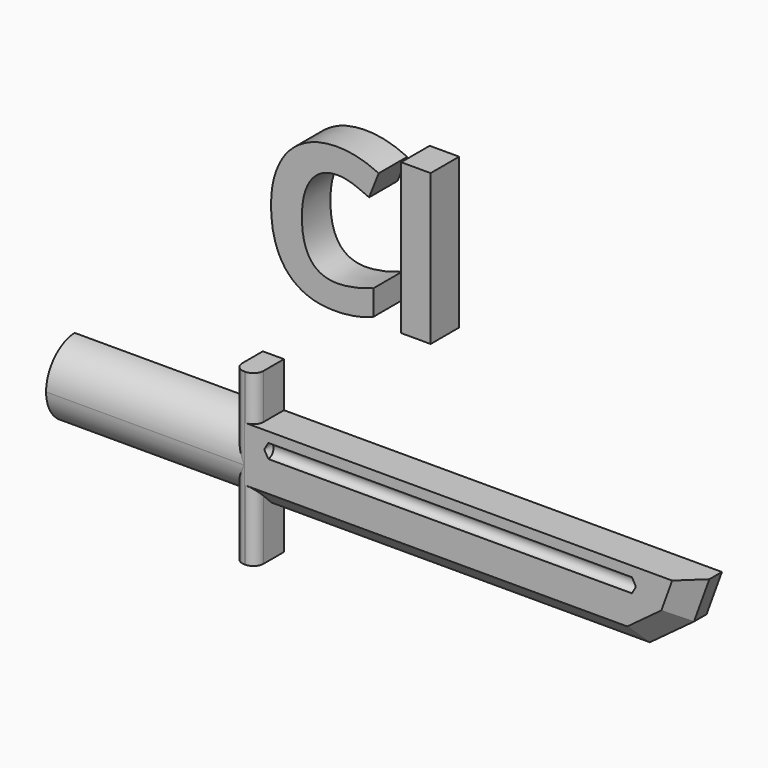
from build123d import *

# Parameters (mm, degrees)
F0_W         = 33.5415452719
F0_H         = 13.3481640369
F0_TEXT_SIZE = 35.2777777778
F1_DEPTH     = 6.35
F2_T1_DEPTH  = 50.2216307033
F3_SIZE      = 3.556
F5_D         = 2.54
F5_DEPTH     = 50.8
F5_TIP       = 0.7630929862
F6_D         = 2.54
F6_DEPTH     = 13.97
F6_TIP       = 0.7630929862
F7_R         = 1.778


# Not quite as in the source:
# - a fillet or chamfer that OpenCascade refuses, or shapes differently, is made with other operations: its cross-section is extruded or revolved along the edge and cut away or added
# - Text() gives the source's letters only with a copy of the font that has no kerning and outlines rounded to 1/6400 em; it was checked with that copy


with BuildPart() as f1:
    # F0 (on Front) → F1 (new body)
    with BuildSketch(Plane.XZ):
        with Locations((-36.8084944785, -14.685629867)):
            Rectangle(F0_W, F0_H)
        Polygon((-20.0377218425, 0), (-20.0377218425, -8.0115478486), (-20.0377218425, -21.3597118855), (-20.0377218425, -30.2584897727), (-16.2728521973, -30.2584897727), (-16.2728521973, -21.3597118855), (-16.2728521973, -11.7764146999), (-16.2728521973, -8.0115478486), (-16.2728521973, 0), align=None)
        Polygon((61.7625713348, -8.0115478486), (-16.2728521973, -8.0115478486), (-16.2728521973, -11.7764146999), (-16.2728521973, -21.3597118855), (51.1524938047, -21.3597118855), (59.0244866908, -15.5412824824), align=None)
        with Locations((-15.5450733329, 15.102172393)):
            Text('Cl', F0_TEXT_SIZE, font='Open Sans', font_style=FontStyle.BOLD, text_align=(TextAlign.LEFT, TextAlign.BOTTOM))
    extrude(amount=F1_DEPTH)

    # F2: fillet of radius 6.6802 on 2 edges, made by hand

    # F2_s2 → F2_t1 (cut)
    with BuildSketch(Plane.YZ.offset(-70.2593525458)):
        with BuildLine():
            ThreePointArc((0, -21.3597118855), (-4.5087499935, -19.2930696615), (-6.35, -14.6876777129))
            Line((-6.35, -14.6876777129), (-6.35, -21.3597118855))
            Line((-6.35, -21.3597118855), (0, -21.3597118855))
        make_face()
        with BuildLine():
            ThreePointArc((0, -8.0115478486), (-4.5087499935, -10.0781900726), (-6.35, -14.6835820212))
            Line((-6.35, -14.6835820212), (-6.35, -8.0115478486))
            Line((-6.35, -8.0115478486), (0, -8.0115478486))
        make_face()
    extrude(amount=F2_T1_DEPTH, mode=Mode.SUBTRACT)

    # F3
    f3_edges = [f1.edges().sort_by_distance(p)[0] for p in [
        (17.439821, -6.35, -21.359712),
        (55.08849, -6.35, -18.450497),
        (60.393529, -6.35, -11.776415),
    ]]
    chamfer(f3_edges, length=F3_SIZE)

    # F5 (one way)
    with BuildSketch(Plane(origin=(0, 0, 0), x_dir=(0, 1, 0), z_dir=(-1, 0, 0))):
        with Locations((-6.4756288193, 11.0805211589)):
            Circle(F5_D / 2)
    extrude(amount=-F5_DEPTH, mode=Mode.SUBTRACT)
    with Locations(Plane(origin=(0, 0, 0), x_dir=(0, 1, 0), z_dir=(-1, 0, 0))):
        with Locations((-6.4756288193, 11.0805211589)):
            with Locations((0, 0, -(F5_DEPTH + F5_TIP / 2))):  # 118° drill point
                Cone(0, F5_D / 2, F5_TIP, mode=Mode.SUBTRACT)

    # F6 (one way)
    with BuildSketch(Plane.YZ):
        with Locations((-6.4756288193, -11.0805211589)):
            Circle(F6_D / 2)
    extrude(amount=-F6_DEPTH, mode=Mode.SUBTRACT)
    with Locations(Plane.YZ):
        with Locations((-6.4756288193, -11.0805211589)):
            with Locations((0, 0, -(F6_DEPTH + F6_TIP / 2))):  # 118° drill point
                Cone(0, F6_D / 2, F6_TIP, mode=Mode.SUBTRACT)

    # F7
    f7_edges = [f1.edges().sort_by_distance(p)[0] for p in [
        (-16.272852, -6.35, -4.005774),
        (-16.272852, -6.35, -24.031101),
        (-20.037722, -6.35, -7.341791),
        (-20.037722, -6.35, -22.473084),
    ]]
    fillet(f7_edges, radius=F7_R)


solid = f1.part
